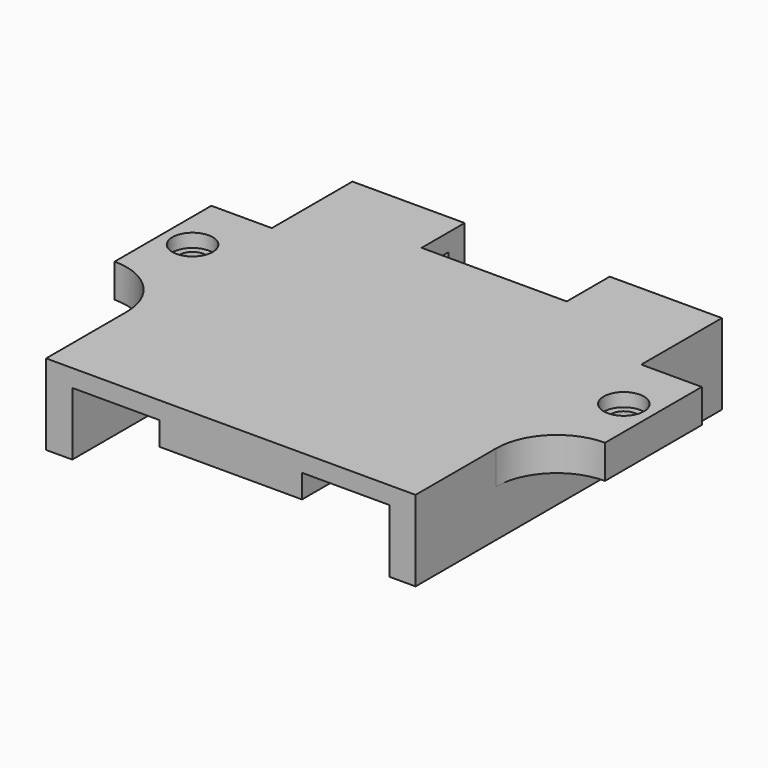
from build123d import *

# Parameters (mm, degrees)
F1_DEPTH       = 28.5
F5_DEPTH       = 2.5
F6_D           = 2
F6_CBORE_D     = 3
F6_CBORE_DEPTH = 1
F7_DEPTH       = 4
F8_W           = 10.6
F8_H           = 5
F9_DEPTH       = 1.75
F3_W           = 6.4
F3_H           = 4.7
F10_DEPTH      = 1.5


# Not quite as in the source:
# - ends of sketch curves that miss each other by under 0.0002 mm in the source are joined


with BuildPart() as f1:
    # F0 (on Front) → F1 (new body)
    with BuildSketch(Plane.XZ):
        Polygon((13.75, 6), (-13.75, 6), (-13.75, 0), (-11.8, 0), (-11.8, 4.7), (11.8, 4.7), (11.8, 0), (13.75, 0), align=None)
    extrude(amount=F1_DEPTH)

    # F4 (on face) → F5 (join)
    with BuildSketch(Plane.XY.offset(6)):
        with BuildLine():
            Line((-13.75, -7.4999997169), (-18.25, -7.4999997169))
            Line((-18.25, -7.4999997169), (-18.25, -16.4999997169))
            ThreePointArc((-18.25, -16.4999997169), (-15.0680194847, -17.8180192015), (-13.75, -20.9999997169))
            Line((-13.75, -20.9999997169), (-13.75, -7.4999997169))
        make_face()
        with BuildLine():
            Line((18.25, -7.4999999106), (13.75, -7.4999999106))
            Line((13.75, -7.4999999106), (13.75, -21))
            ThreePointArc((13.75, -21), (15.0680194847, -17.8180192015), (18.25, -16.4999997169))
            Line((18.25, -16.4999997169), (18.25, -7.4999999106))
        make_face()
    extrude(amount=-F5_DEPTH)

    # F6 (through all)
    with Locations(Plane.XY.offset(6)):
        with Locations((-16.05, -11.9999998212), (16.05, -11.9999998212)):
            CounterBoreHole(F6_D / 2, F6_CBORE_D / 2, F6_CBORE_DEPTH)

    # F3 (on face) → F7 (cut)
    with BuildSketch(Plane(origin=(0, 0, 0), x_dir=(-1, 0, 0), z_dir=(0, 1, 0))):
        Polygon((-5.4, 4.7), (-5.4, 0), (0, 0), (5.4, 0), (5.4, 4.7), (5.4, 6), (-5.4, 6), align=None)
    extrude(amount=-F7_DEPTH, mode=Mode.SUBTRACT)

    # F8 (on face) → F9 (join)
    with BuildSketch(Plane(origin=(0, 0, 4.7), x_dir=(1, 0, 0), z_dir=(0, 0, -1))):
        with Locations((0, 26)):
            Rectangle(F8_W, F8_H)
    extrude(amount=F9_DEPTH)

    # F3 (on face) → F10 (join)
    with BuildSketch(Plane(origin=(0, 0, 0), x_dir=(-1, 0, 0), z_dir=(0, 1, 0))):
        with Locations((-8.6, 2.35)):
            Rectangle(F3_W, F3_H)
        with Locations((8.6, 2.35)):
            Rectangle(F3_W, F3_H)
    extrude(amount=-F10_DEPTH)


solid = f1.part
